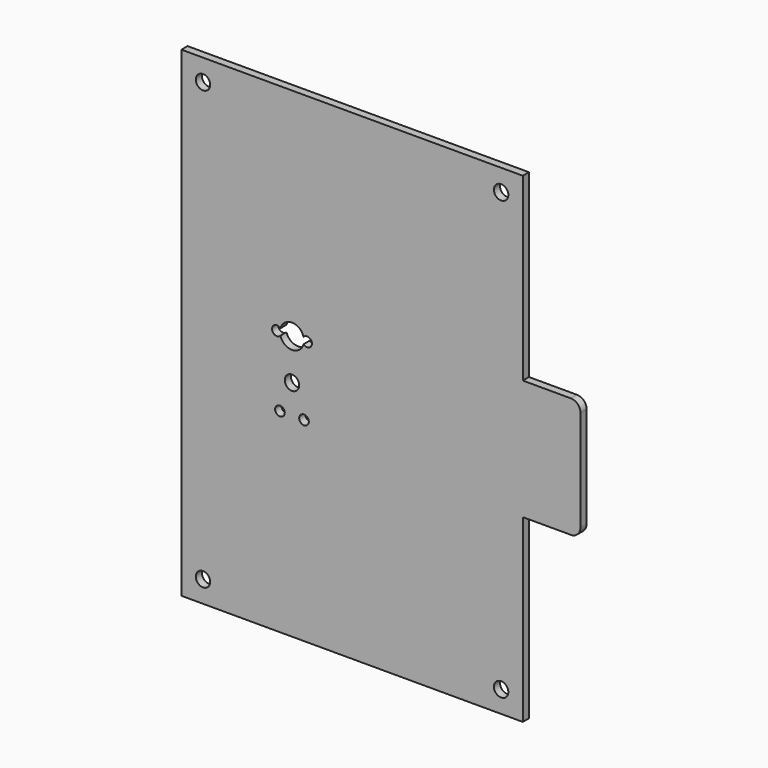
from build123d import *

# Parameters (mm, degrees)
F0_R     = 1.5
F0_R_2   = 1
F1_DEPTH = 1.6


with BuildPart() as f1:
    # F0 (on Front) → F1 (new body)
    with BuildSketch(Plane.XZ):
        with BuildLine():
            Line((35.5, 50), (-35.5, 50))
            Line((-35.5, 50), (-35.5, 35))
            Line((-35.5, 35), (-35.5, -27))
            Line((-35.5, -27), (-35.5, -50))
            Line((-35.5, -50), (35.5, -50))
            Line((35.5, -50), (35.5, -12.5))
            Line((35.5, -12.5), (45.5, -12.5))
            ThreePointArc((45.5, -12.5), (46.9142135624, -11.9142135624), (47.5, -10.5))
            Line((47.5, -10.5), (47.5, 10.5))
            ThreePointArc((47.5, 10.5), (46.9142135624, 11.9142135624), (45.5, 12.5))
            Line((45.5, 12.5), (35.5, 12.5))
            Line((35.5, 12.5), (35.5, 50))
        make_face()
        with Locations((-31, -45.5)):
            Circle(F0_R, mode=Mode.SUBTRACT)
        with Locations((-15, -9.5)):
            Circle(F0_R_2, mode=Mode.SUBTRACT)
        with Locations((-10, -9.5)):
            Circle(F0_R_2, mode=Mode.SUBTRACT)
        with Locations((-12.5, -3.5)):
            Circle(F0_R, mode=Mode.SUBTRACT)
        with Locations((31, -45.5)):
            Circle(F0_R, mode=Mode.SUBTRACT)
        with BuildLine():
            ThreePointArc((-12.5, 7.5), (-10.9878693139, 6.99084424), (-10.0916666667, 5.6707686304))
            ThreePointArc((-10.0916666667, 5.6707686304), (-8.9906023558, 5.9331845119), (-8.35, 5))
            ThreePointArc((-8.35, 5), (-8.9906023558, 4.0668154881), (-10.0916666667, 4.3292313696))
            ThreePointArc((-10.0916666667, 4.3292313696), (-12.5, 2.5), (-14.9083333333, 4.3292313696))
            ThreePointArc((-14.9083333333, 4.3292313696), (-16.65, 5), (-14.9083333333, 5.6707686304))
            ThreePointArc((-14.9083333333, 5.6707686304), (-14.0121306861, 6.99084424), (-12.5, 7.5))
        make_face(mode=Mode.SUBTRACT)
        with Locations((-31, 45.5)):
            Circle(F0_R, mode=Mode.SUBTRACT)
        with Locations((31, 45.5)):
            Circle(F0_R, mode=Mode.SUBTRACT)
    extrude(amount=-F1_DEPTH)


solid = f1.part
